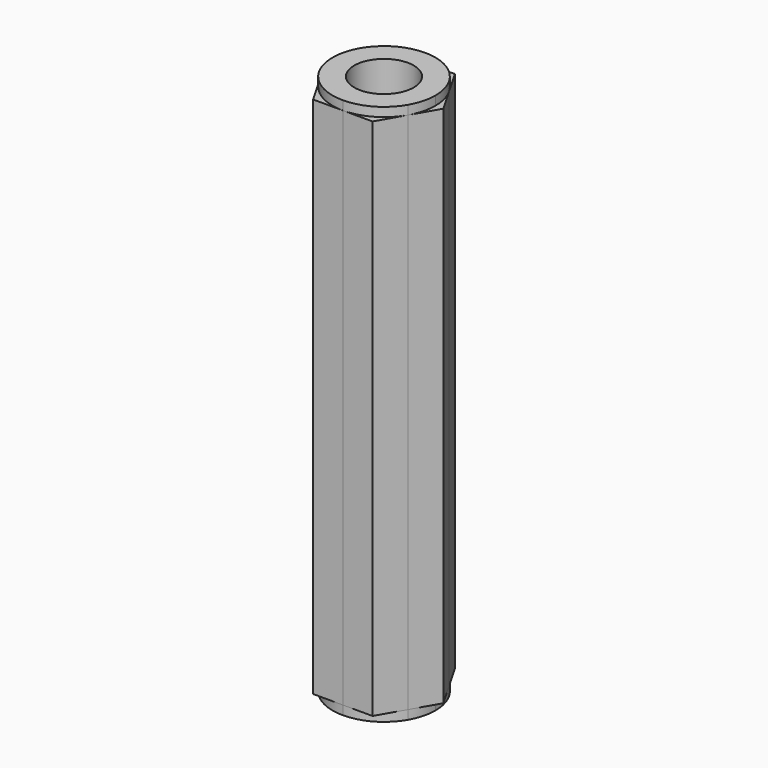
from build123d import *

# Parameters (mm, degrees)
F2_DEPTH = 14.5
F0_R     = 1.65
F3_DEPTH = 15


# Not quite as in the source:
# - the program builds the solid bodies; features that only make, move or delete a surface that nothing else refers to are left out


with BuildPart() as f2:
    # F0 (on Top) → F2 (new body, symmetric)
    with BuildSketch(Plane.XY):
        with BuildLine():
            ThreePointArc((-2.4681723606, -1.4250000696), (-2.85, -3.73e-08), (-2.4681723979, 1.425000005))
            Line((-2.4681723979, 1.425000005), (-3.2908965344, 0))
            Line((-3.2908965344, 0), (-2.4681723606, -1.4250000696))
        make_face()
    extrude(amount=F2_DEPTH, both=True)



with BuildPart() as f2b:
    # F0 (on Top) → F2, piece 2 (new body, symmetric)
    with BuildSketch(Plane.XY):
        with BuildLine():
            ThreePointArc((-2.4681723979, 1.425000005), (-1.4249999975, 2.4681724022), (0, 2.85))
            Line((0, 2.85), (-1.6454482672, 2.85))
            Line((-1.6454482672, 2.85), (-2.4681723979, 1.425000005))
        make_face()
    extrude(amount=F2_DEPTH, both=True)


with BuildPart() as f2c:
    # F0 (on Top) → F2, piece 3 (new body, symmetric)
    with BuildSketch(Plane.XY):
        with BuildLine():
            ThreePointArc((0, 2.85), (1.4249999814, 2.4681724115), (2.4681723793, 1.4250000373))
            Line((2.4681723793, 1.4250000373), (1.6454482672, 2.85))
            Line((1.6454482672, 2.85), (0, 2.85))
        make_face()
    extrude(amount=F2_DEPTH, both=True)


with BuildPart() as f2d:
    # F0 (on Top) → F2, piece 4 (new body, symmetric)
    with BuildSketch(Plane.XY):
        with BuildLine():
            ThreePointArc((2.4681723793, 1.4250000373), (2.7528885994, 0.7376342993), (2.85, 0))
            ThreePointArc((2.85, 0), (2.7528886042, -0.7376342813), (2.4681723979, -1.425000005))
            Line((2.4681723979, -1.425000005), (3.2908965344, 0))
            Line((3.2908965344, 0), (2.4681723793, 1.4250000373))
        make_face()
    extrude(amount=F2_DEPTH, both=True)


with BuildPart() as f2e:
    # F0 (on Top) → F2, piece 5 (new body, symmetric)
    with BuildSketch(Plane.XY):
        with BuildLine():
            Line((1.6454482672, -2.85), (2.4681723979, -1.425000005))
            ThreePointArc((2.4681723979, -1.425000005), (1.4249999975, -2.4681724022), (0, -2.85))
            Line((0, -2.85), (1.6454482672, -2.85))
        make_face()
    extrude(amount=F2_DEPTH, both=True)


with BuildPart() as f2f:
    # F0 (on Top) → F2, piece 6 (new body, symmetric)
    with BuildSketch(Plane.XY):
        with BuildLine():
            Line((-1.6454482672, -2.85), (0, -2.85))
            ThreePointArc((0, -2.85), (-1.4249999652, -2.4681724209), (-2.4681723606, -1.4250000696))
            Line((-2.4681723606, -1.4250000696), (-1.6454482672, -2.85))
        make_face()
    extrude(amount=F2_DEPTH, both=True)


with BuildPart() as f2_1:
    add(f2.part)

    add(f2b.part)  # F3 merges F2b

    add(f2c.part)  # F3 merges F2c

    add(f2d.part)  # F3 merges F2d

    add(f2e.part)  # F3 merges F2e

    add(f2f.part)  # F3 merges F2f
    # F0 (on Top) → F3 (join, symmetric)
    with BuildSketch(Plane.XY):
        with BuildLine():
            ThreePointArc((2.4681723979, -1.425000005), (2.7528886042, -0.7376342813), (2.85, 0))
            ThreePointArc((2.85, 0), (2.7528885994, 0.7376342993), (2.4681723793, 1.4250000373))
            ThreePointArc((2.4681723793, 1.4250000373), (1.4249999814, 2.4681724115), (0, 2.85))
            ThreePointArc((0, 2.85), (-1.4249999975, 2.4681724022), (-2.4681723979, 1.425000005))
            ThreePointArc((-2.4681723979, 1.425000005), (-2.85, -3.73e-08), (-2.4681723606, -1.4250000696))
            ThreePointArc((-2.4681723606, -1.4250000696), (-1.4249999652, -2.4681724209), (0, -2.85))
            ThreePointArc((0, -2.85), (1.4249999975, -2.4681724022), (2.4681723979, -1.425000005))
        make_face()
        Circle(F0_R, mode=Mode.SUBTRACT)
    extrude(amount=F3_DEPTH, both=True)


solid = f2_1.part
